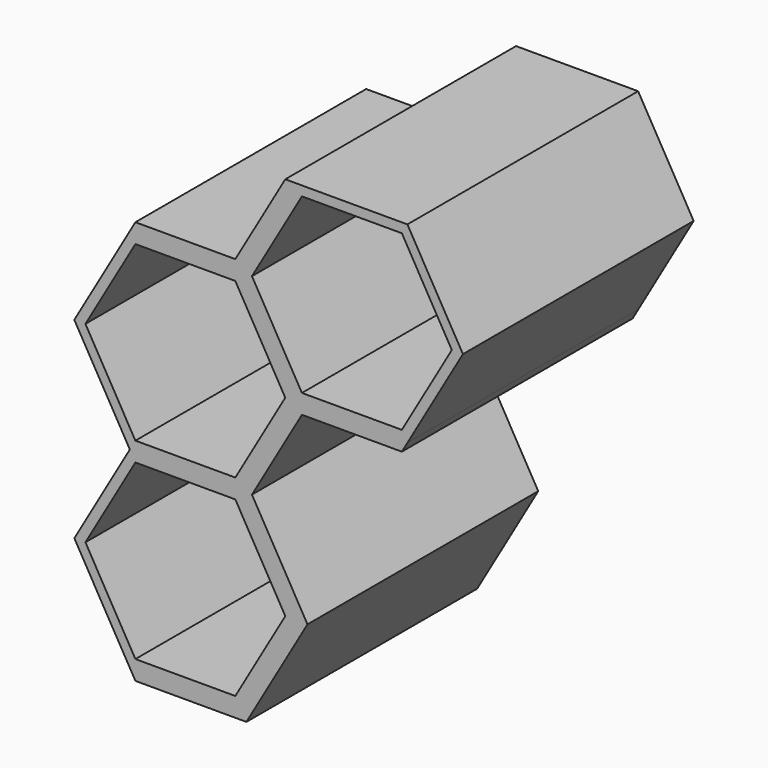
from build123d import *

# Parameters (mm, degrees)
F1_DEPTH = 12.7
F2_DEPTH = 95.25


# Not quite as in the source:
# - a feature names something its author has since deleted; it is built from what else it names


with BuildPart() as f1:
    # F0 (on Front) → F1 (new body)
    with BuildSketch(Plane.XZ):
        Polygon((-4.278267482, -28.4575006988), (-22.6091385288, 3.2924993012), (-59.2708806223, 3.2924993012), (-77.6017516691, -28.4575006988), (-59.2708806223, -60.2075006988), (-22.6091385288, -60.2075006988), align=None)
        Polygon((-57.4377935176, -57.0325006988), (-73.9355774597, -28.4575006988), (-57.4377935176, 0.1174993012), (-24.4422256334, 0.1174993012), (-7.9444416913, -28.4575006988), (-24.4422256334, -57.0325006988), align=None, mode=Mode.SUBTRACT)
        Polygon((-22.6091385288, 3.2924993012), (-4.278267482, 35.0424993012), (-22.6091385288, 66.7924993012), (-27.4963065598, 66.7924993012), (-59.2708806223, 66.7924993012), (-77.6017516691, 35.0424993012), (-59.2708806223, 3.2924993012), align=None)
        Polygon((-57.4377935176, 6.4674993012), (-73.9355774597, 35.0424993012), (-57.4377935176, 63.6174993012), (-24.4422256334, 63.6174993012), (-7.9444416913, 35.0424993012), (-24.4422256334, 6.4674993012), align=None, mode=Mode.SUBTRACT)
        Polygon((-22.6091385288, 66.7924993012), (-4.278267482, 35.0424993012), (27.4963065701, 35.0424993012), (32.3834746115, 35.0424993012), (50.7143456583, 66.7924993012), (32.3834746115, 98.5424993012), (-4.278267482, 98.5424993012), align=None)
        Polygon((-2.4451803773, 38.2174993012), (-18.9429643194, 66.7924993012), (-2.4451803773, 95.3674993012), (30.5503875069, 95.3674993012), (47.048171449, 66.7924993012), (30.5503875069, 38.2174993012), align=None, mode=Mode.SUBTRACT)
        Polygon((-2.4451803773, 95.3674993012), (-18.9429643194, 66.7924993012), (-2.4451803773, 38.2174993012), (30.5503875069, 38.2174993012), (47.048171449, 66.7924993012), (30.5503875069, 95.3674993012), align=None)
        Polygon((-57.4377935176, 0.1174993012), (-73.9355774597, -28.4575006988), (-57.4377935176, -57.0325006988), (-24.4422256334, -57.0325006988), (-7.9444416913, -28.4575006988), (-24.4422256334, 0.1174993012), align=None)
        Polygon((-57.4377935176, 63.6174993012), (-73.9355774597, 35.0424993012), (-57.4377935176, 6.4674993012), (-24.4422256334, 6.4674993012), (-7.9444416913, 35.0424993012), (-24.4422256334, 63.6174993012), align=None)
    extrude(amount=F1_DEPTH)

    # F0 (on Front) → F2 (join)
    with BuildSketch(Plane.XZ):
        Polygon((-22.6091385288, 3.2924993012), (-4.278267482, 35.0424993012), (-22.6091385288, 66.7924993012), (-27.4963065598, 66.7924993012), (-59.2708806223, 66.7924993012), (-77.6017516691, 35.0424993012), (-59.2708806223, 3.2924993012), align=None)
        Polygon((-57.4377935176, 6.4674993012), (-73.9355774597, 35.0424993012), (-57.4377935176, 63.6174993012), (-24.4422256334, 63.6174993012), (-7.9444416913, 35.0424993012), (-24.4422256334, 6.4674993012), align=None, mode=Mode.SUBTRACT)
        Polygon((-22.6091385288, 66.7924993012), (-4.278267482, 35.0424993012), (27.4963065701, 35.0424993012), (32.3834746115, 35.0424993012), (50.7143456583, 66.7924993012), (32.3834746115, 98.5424993012), (-4.278267482, 98.5424993012), align=None)
        Polygon((-2.4451803773, 38.2174993012), (-18.9429643194, 66.7924993012), (-2.4451803773, 95.3674993012), (30.5503875069, 95.3674993012), (47.048171449, 66.7924993012), (30.5503875069, 38.2174993012), align=None, mode=Mode.SUBTRACT)
        Polygon((-4.278267482, -28.4575006988), (-22.6091385288, 3.2924993012), (-59.2708806223, 3.2924993012), (-77.6017516691, -28.4575006988), (-59.2708806223, -60.2075006988), (-22.6091385288, -60.2075006988), align=None)
        Polygon((-57.4377935176, -57.0325006988), (-73.9355774597, -28.4575006988), (-57.4377935176, 0.1174993012), (-24.4422256334, 0.1174993012), (-7.9444416913, -28.4575006988), (-24.4422256334, -57.0325006988), align=None, mode=Mode.SUBTRACT)
        Polygon((27.4963065701, 35.0424993012), (-4.278267482, 35.0424993012), (-22.6091385288, 3.2924993012), (-4.278267482, -28.4575006988), (-22.6091385288, -60.2075006988), (-59.2708806223, -60.2075006988), (-57.4378374826, -63.3825006988), (-20.7760404334, -63.3825006988), (-0.612082282, -28.4575006988), (-18.9429533288, 3.2924993012), (-2.4451693867, 31.8674993012), (30.5503875069, 31.8674993012), (32.3834746115, 35.0424993012), align=None)
        Polygon((-27.4963065598, 66.7924993012), (-22.6091385288, 66.7924993012), (-4.278267482, 98.5424993012), (-7.9444416913, 98.5424993012), (-24.4422256334, 69.9674993012), (-57.4377935176, 69.9674993012), (-59.2708806223, 66.7924993012), align=None)
    extrude(amount=F2_DEPTH)


solid = f1.part
